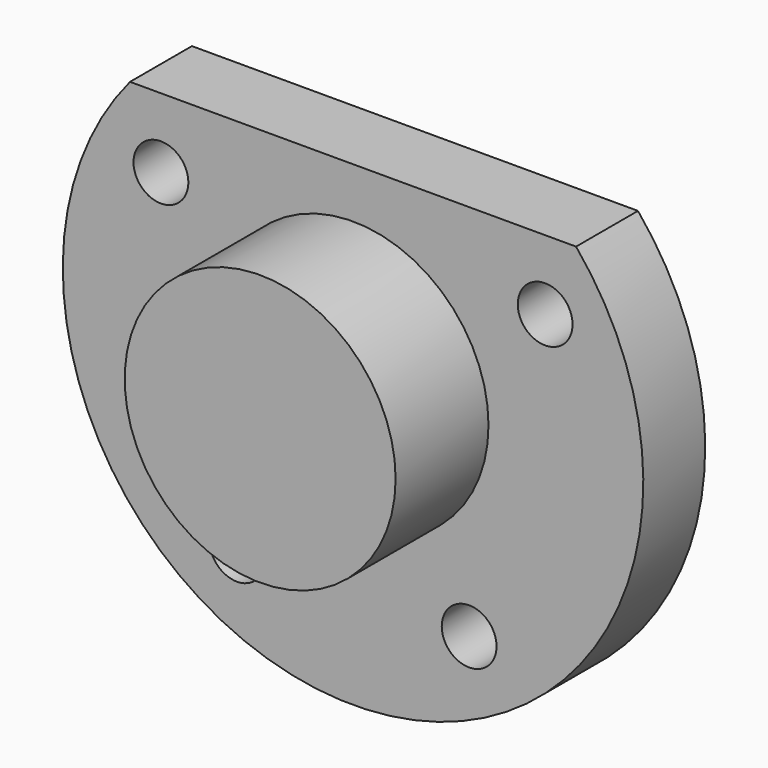
from build123d import *

# Parameters (mm, degrees)
F1_DEPTH = 6.35
F3_D     = 4.4958
F4_R     = 11.1125
F5_DEPTH = 9.525


with BuildPart() as f1:
    # F0 (on Front) → F1 (new body)
    with BuildSketch(Plane.XZ):
        with BuildLine():
            Line((18.2969275085, 15.24), (-18.2969275085, 15.24))
            ThreePointArc((-18.2969275085, 15.24), (0, -23.8125), (18.2969275085, 15.24))
        make_face()
    extrude(amount=F1_DEPTH)

    # F3 (through all)
    with Locations(Plane.XZ.offset(6.35)):
        with Locations((-9.525, -15.7602855304), (-15.7602855304, 9.525), (15.7602855304, 9.525), (9.525, -15.7602855304)):
            Hole(F3_D / 2)

    # F4 (on face) → F5 (join)
    with BuildSketch(Plane.XZ.offset(6.35)):
        Circle(F4_R)
    extrude(amount=F5_DEPTH)


solid = f1.part
